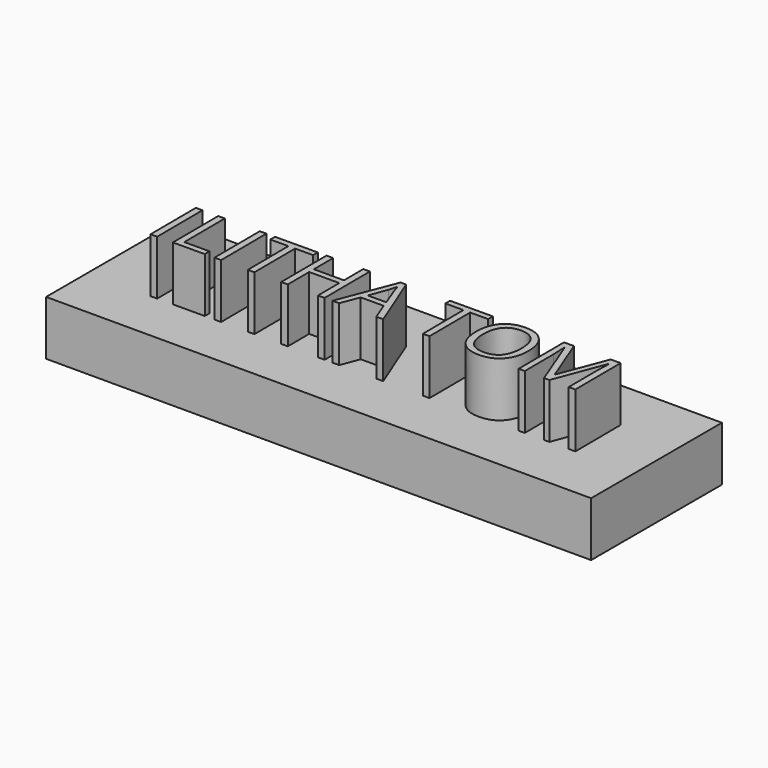
from build123d import *

# Parameters (mm, degrees)
F0_W         = 50
F0_H         = 15
F1_DEPTH     = 5
F2_TEXT_SIZE = 7.3228639263
F3_DEPTH     = 5


# Not quite as in the source:
# - Text() gives the source's letters only with a copy of the font that has no kerning and outlines rounded to 1/6400 em; it was checked with that copy


with BuildPart() as f1:
    # F0 (on Top) → F1 (new body)
    with BuildSketch(Plane.XY):
        with Locations((25, 7.5)):
            Rectangle(F0_W, F0_H)
    extrude(amount=F1_DEPTH)

    # F2 (on face) → F3 (join)
    with BuildSketch(Plane.XY.offset(5)):
        with Locations(Location((5.0558564947, 4.7549138022), (0, 0, 0.3119606169))):
            Text('ILITHA TOM', F2_TEXT_SIZE, font='Open Sans', text_align=(TextAlign.LEFT, TextAlign.BOTTOM))
    extrude(amount=F3_DEPTH)


solid = f1.part
